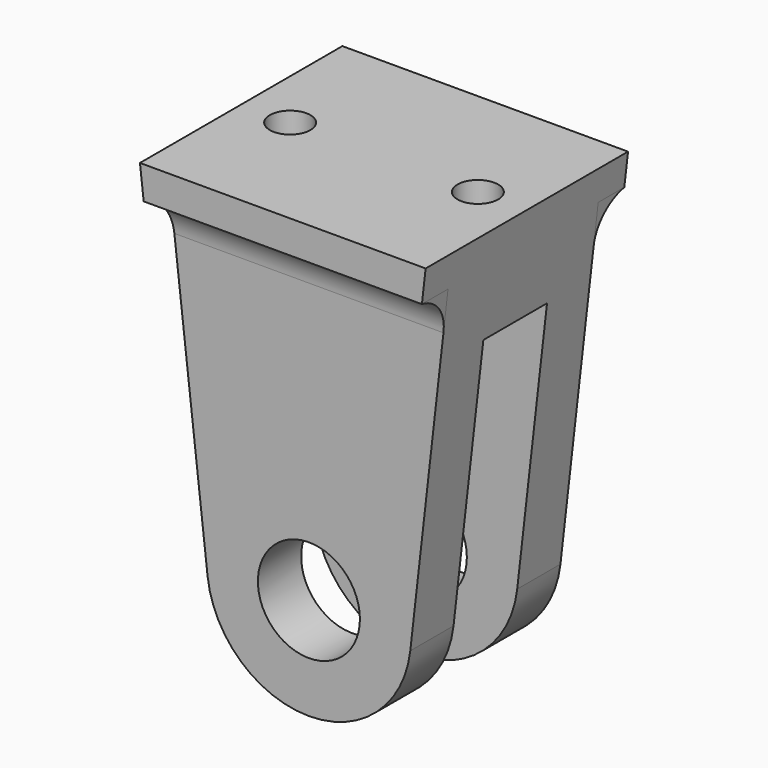
from build123d import *

# Parameters (mm, degrees)
F0_R         = 3.175
F1_DEPTH     = 15.748
F2_W         = 4.953
F2_H         = 16.2648302115
F2_H_2       = 7.994236929
F3_DEPTH     = 12.7
F2_W_2       = 2.032
F2_H_3       = 20.5828301237
F4_DEPTH     = 12.7
F5_T4_DEPTH  = 29.7595972634
F5_T10_DEPTH = 29.7595972634
F7_D         = 2.5273


# Not quite as in the source:
# - a fillet or chamfer that OpenCascade refuses, or shapes differently, is made with other operations: its cross-section is extruded or revolved along the edge and cut away or added


with BuildPart() as f1:
    # F0 (on Front) → F1 (new body)
    with BuildSketch(Plane.XZ):
        with BuildLine():
            Line((-8.89, 21.8948), (-6.3090456189, -0.7200301237))
            ThreePointArc((-6.3090456189, -0.7200301237), (0, -6.35), (6.3090456189, -0.7200301237))
            Line((6.3090456189, -0.7200301237), (8.89, 21.8948))
            Line((8.89, 21.8948), (-8.89, 21.8948))
        make_face()
        Circle(F0_R, mode=Mode.SUBTRACT)
    extrude(amount=F1_DEPTH)

    # F2 (on Right) → F3 (cut, symmetric)
    with BuildSketch(Plane.YZ):
        with Locations((-7.874, 7.4123849821)):
            Rectangle(F2_W, F2_H)
        with Locations((-7.874, -4.7171485882)):
            Rectangle(F2_W, F2_H_2)
    extrude(amount=F3_DEPTH, both=True, mode=Mode.SUBTRACT)

    # F2 (on Right) → F4 (cut, symmetric)
    with BuildSketch(Plane.YZ):
        with Locations((-14.732, -4.7171485882)):
            Rectangle(F2_W_2, F2_H_2)
        with Locations((-1.016, -4.7171485882)):
            Rectangle(F2_W_2, F2_H_2)
        with Locations((-1.016, 9.5713849382)):
            Rectangle(F2_W_2, F2_H_3)
        with Locations((-14.732, 9.5713849382)):
            Rectangle(F2_W_2, F2_H_3)
    extrude(amount=F4_DEPTH, both=True, mode=Mode.SUBTRACT)

    # F5: fillet of radius 2.54 on 2 edges, made by hand


with BuildPart() as f5_tool2:
    # F5_s3 → F5_t4 (new body)
    with BuildSketch(Plane.YZ.offset(-14.8797986317)):
        with BuildLine():
            ThreePointArc((-15.748, 19.8628), (-14.2885244601, 18.9805554727), (-13.716, 17.3741184213))
            Line((-13.716, 17.3741184213), (-13.716, 19.8628))
            Line((-13.716, 19.8628), (-15.748, 19.8628))
        make_face()
    extrude(amount=F5_T4_DEPTH)

    split(bisect_by=Plane(origin=(6.3090456189, 0, -0.7200301237), x_dir=(0, 1, 0), z_dir=(-0.9935504912, 0, 0.1133905707)), keep=Keep.TOP)

    split(bisect_by=Plane(origin=(-6.3090456189, 0, -0.7200301237), x_dir=(0, 1, 0), z_dir=(0.9935504912, 0, 0.1133905707)), keep=Keep.TOP)


with BuildPart() as f1_1:
    add(f1.part)

    # F5_t1: union F5_tool2
    add(f5_tool2.part)


with BuildPart() as f5_tool8:
    # F5_s9 → F5_t10 (new body)
    with BuildSketch(Plane.YZ.offset(14.8797986317)):
        with BuildLine():
            ThreePointArc((-2.032, 17.3741184213), (-1.4594755399, 18.9805554727), (0, 19.8628))
            Line((0, 19.8628), (-2.032, 19.8628))
            Line((-2.032, 19.8628), (-2.032, 17.3741184213))
        make_face()
    extrude(amount=-F5_T10_DEPTH)

    split(bisect_by=Plane(origin=(6.3090456189, 0, -0.7200301237), x_dir=(0, 1, 0), z_dir=(-0.9935504912, 0, 0.1133905707)), keep=Keep.TOP)

    split(bisect_by=Plane(origin=(-6.3090456189, 0, -0.7200301237), x_dir=(0, 1, 0), z_dir=(0.9935504912, 0, 0.1133905707)), keep=Keep.TOP)


with BuildPart() as f1_2:
    add(f1_1.part)

    # F5_t7: union F5_tool8
    add(f5_tool8.part)

    # F7 (through all)
    with Locations(Plane.XY.offset(21.8948)):
        with Locations((-5.842, -7.874), (5.842, -7.874)):
            Hole(F7_D / 2)


solid = f1_2.part
